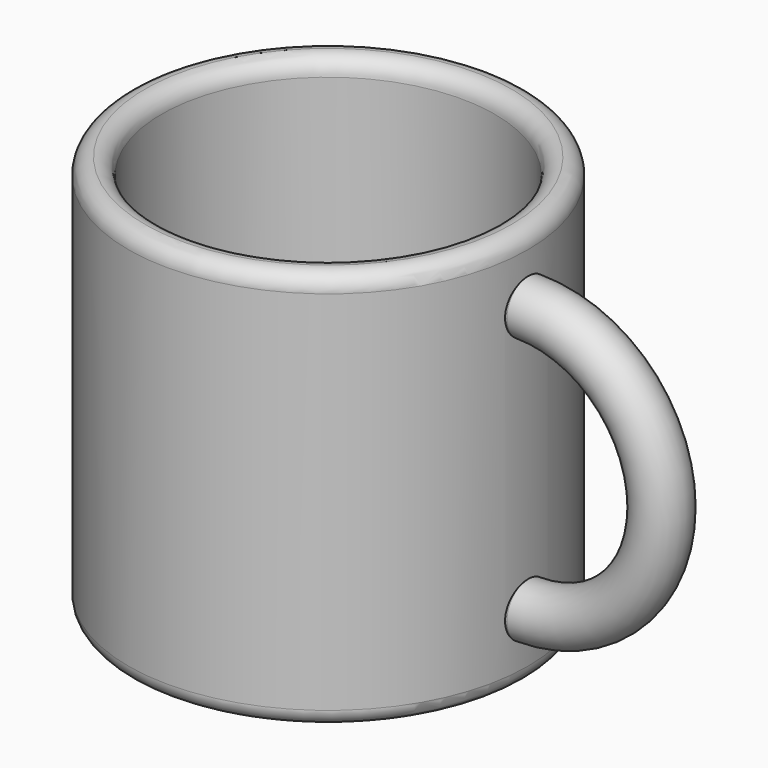
from build123d import *
from build123d import SkipClean  # not in build123d's __all__

# Parameters (mm, degrees)
F0_W      = 19.05
F0_H      = 38.1
F2_R      = 15.875
F3_DEPTH  = 34.925
F6_R      = 1.58749
F7_R      = 1.5875
F8_R      = 2.54
F10_R     = 2.54
F11_R     = 2.54
F12_DEPTH = 3.175


# Not quite as in the source:
# - a fillet or chamfer is up to 0.001 mm smaller than in the source, because OpenCascade refuses the exact size


with BuildPart() as f1:
    # F0 (on Front) → F1 (revolve)
    with BuildSketch(Plane.XZ):
        with Locations((9.525, 19.05)):
            Rectangle(F0_W, F0_H)
    revolve(axis=Axis((0, 0, 19.05), (0, 0, 1)))

    # F2 (on face) → F3 (cut)
    with BuildSketch(Plane.XY.offset(38.1)):
        Circle(F2_R)
    extrude(amount=-F3_DEPTH, mode=Mode.SUBTRACT)

    # F6 (radius 1.5875 in the source; OpenCascade refuses exactly that, so slightly less here)
    f6_edges = [f1.edges().sort_by_distance(p)[0] for p in [
        (-19.05, 0, 38.1),
        (-15.875, 0, 38.1),
    ]]
    fillet(f6_edges, radius=F6_R)

    # F7
    f7_edges = [f1.edges().sort_by_distance(p)[0] for p in [
        (-19.05, 0, 0),
    ]]
    fillet(f7_edges, radius=F7_R)

    # F9: sweep along a path in F5
    with BuildLine(Plane.XZ) as f9_path:
        ThreePointArc((19.05, 6.35), (31.75, 19.05), (19.05, 31.75))
    # F8 (on offset) → F9 (sweep)
    with BuildSketch(Plane.YZ.offset(19.05)):
        with Locations((0, 31.75)):
            Circle(F8_R)
    sweep(path=f9_path.line)

    # F10 (on face) + F11 (on face) → F12 (join, through all)
    with BuildSketch(Plane(origin=(19.05, 0, 0), x_dir=(0, -1, 0), z_dir=(-1, 0, 0))):
        with Locations((0, 31.75)):
            Circle(F10_R)
    with BuildSketch(Plane(origin=(19.05, 0, 0), x_dir=(0, -1, 0), z_dir=(-1, 0, 0))):
        with Locations((0, 6.35)):
            Circle(F11_R)
    with SkipClean():  # cleaning this boolean's faces spoils the solid; the shape is the same uncleaned
        extrude(amount=F12_DEPTH)


solid = f1.part
